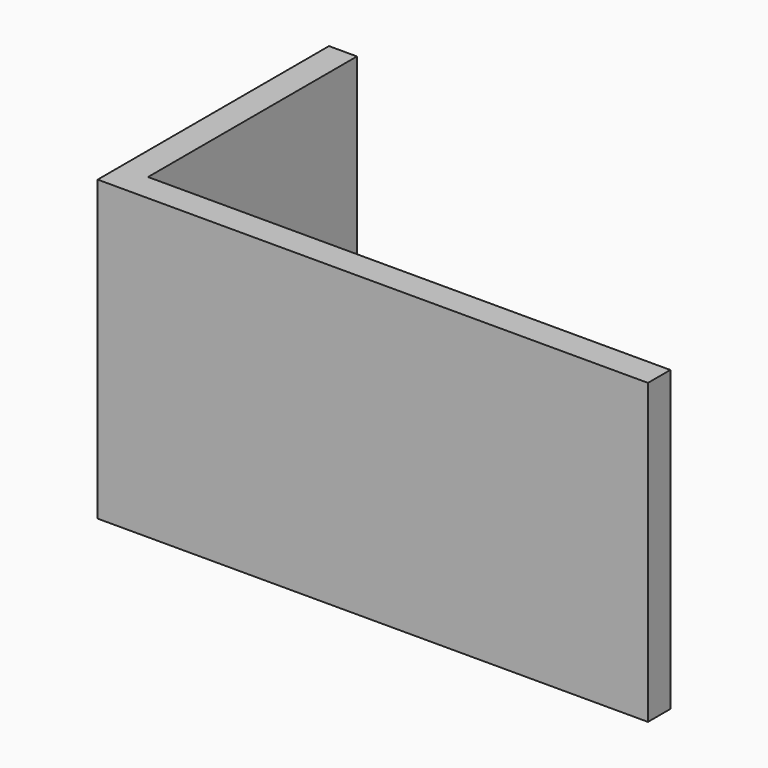
from build123d import *

# Parameters (mm, degrees)
F1_DEPTH = 3200


# Not quite as in the source:
# - a feature of the source that left no trace in its solid (it failed there, or was rolled back) is left out


with BuildPart() as f1:
    # F0 (on Top) → F1 (new body)
    with BuildSketch(Plane.XY):
        Polygon((0, -300), (0, 0), (-5600, 0), (-5600, 2800), (-5900, 2800), (-5900, -300), align=None)
    extrude(amount=F1_DEPTH)


solid = f1.part
